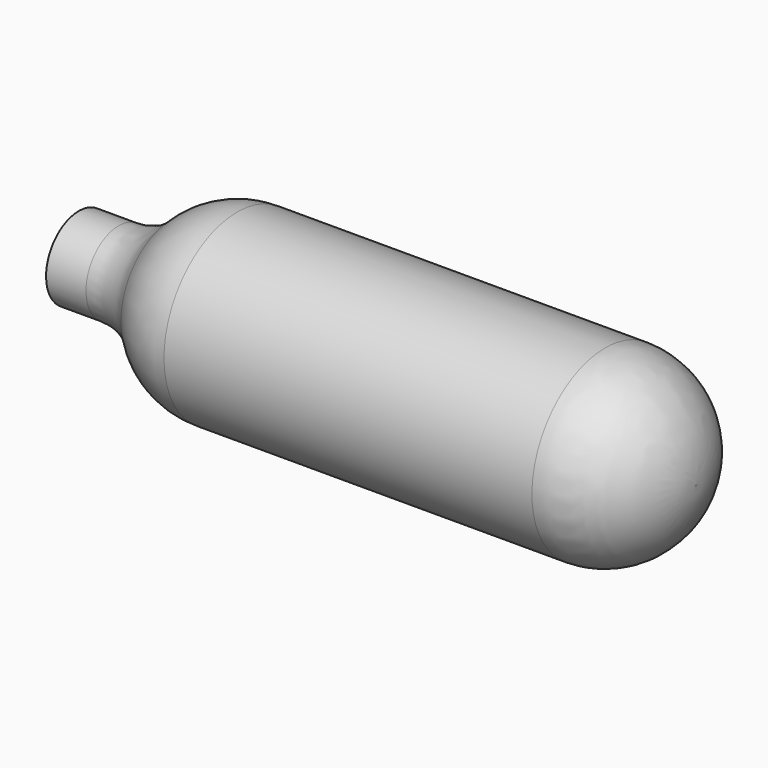
from build123d import *

# Parameters (mm, degrees)
F2_R     = 9.398
F4_R     = 7.62
F5_R     = 0.9906
F6_DEPTH = 25.4


# Not quite as in the source:
# - a fillet or chamfer that OpenCascade refuses, or shapes differently, is made with other operations: its cross-section is extruded or revolved along the edge and cut away or added


with BuildPart() as f1:
    # F0 (on Front) → F1 (revolve)
    with BuildSketch(Plane.XZ):
        Polygon((-32.9808058875, 0), (0, 0), (31.0198143902, 0), (31.0271941125, 9.4996), (-24.9798058875, 9.4996), (-24.9798058875, 4.2418), (-32.9808058875, 4.2418), align=None)
    revolve(axis=Axis((15.5099071951, 0, 0), (1, 0, 0)))

    # F2
    f2_edges = [f1.edges().sort_by_distance(p)[0] for p in [
        (31.027194, 0, -9.4996),
        (31.023504, 0, 4.7498),
    ]]
    fillet(f2_edges, radius=F2_R)

    # F3: fillet of radius 9.398 on 1 edges, made by hand

    # F3_s1 → F3_t2 (revolve, cut)
    with BuildSketch(Plane.XZ):
        with BuildLine():
            ThreePointArc((-16.542913808, 9.4996), (-21.5134673185, 8.0775640044), (-24.9798058875, 4.2418))
            Line((-24.9798058875, 4.2418), (-24.9798058875, 9.4996))
            Line((-24.9798058875, 9.4996), (-16.542913808, 9.4996))
        make_face()
    revolve(axis=Axis((-24.9798058875, 0, 0), (1, 0, 0)), mode=Mode.SUBTRACT)

    # F4
    f4_edges = [f1.edges().sort_by_distance(p)[0] for p in [
        (-24.979806, 0, -4.2418),
    ]]
    fillet(f4_edges, radius=F4_R)

    # F5 (on face) → F6 (cut)
    with BuildSketch(Plane(origin=(-32.9808058875, 0, 0), x_dir=(0, -1, 0), z_dir=(-1, 0, 0))):
        Circle(F5_R)
    extrude(amount=-F6_DEPTH, mode=Mode.SUBTRACT)


solid = f1.part
